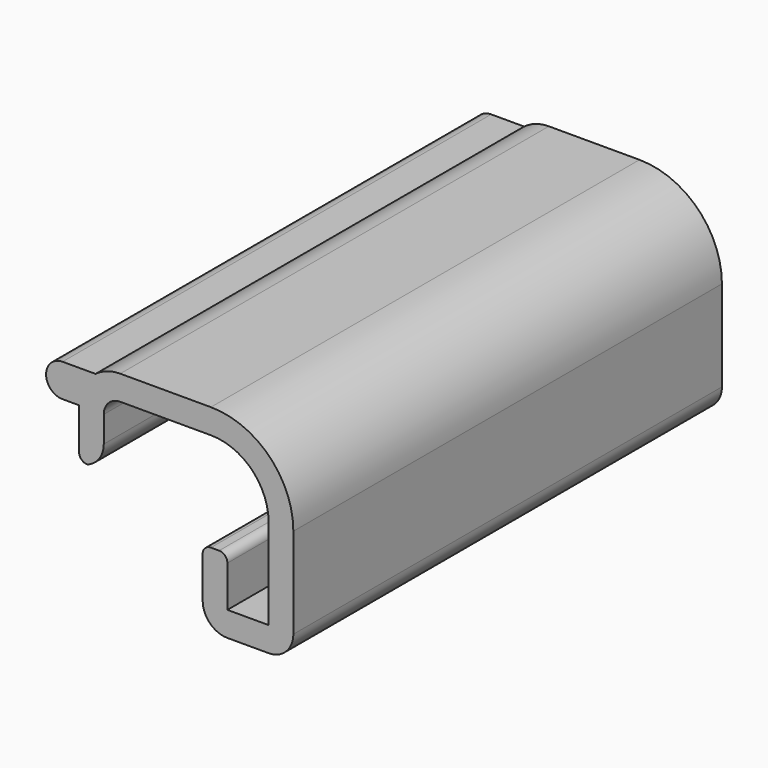
from build123d import *

# Parameters (mm, degrees)
F1_DEPTH    = 65
F2_R        = 1
F3_R        = 1.99999
F4_T1_DEPTH = 79.1421356237


# Not quite as in the source:
# - a fillet or chamfer that OpenCascade refuses, or shapes differently, is made with other operations: its cross-section is extruded or revolved along the edge and cut away or added
# - a fillet or chamfer is up to 0.001 mm smaller than in the source, because OpenCascade refuses the exact size
# - a feature names something its author has since deleted; it is built from what else it names


with BuildPart() as f1:
    # F0 (on Front) → F1 (new body)
    with BuildSketch(Plane.XZ):
        with BuildLine():
            ThreePointArc((0, -2), (0.5857864376, -0.5857864376), (2, 0))
            Line((2, 0), (13, 0))
            ThreePointArc((13, 0), (17.9497474683, -2.0502525317), (20, -7))
            Line((20, -7), (20, -18))
            Line((20, -18), (15, -18))
            Line((15, -18), (15, -12))
            Line((15, -12), (12, -12))
            Line((12, -12), (12, -18))
            ThreePointArc((12, -18), (12.8786796564, -20.1213203436), (15, -21))
            Line((15, -21), (20, -21))
            ThreePointArc((20, -21), (22.1213203436, -20.1213203436), (23, -18))
            Line((23, -18), (23, -7))
            ThreePointArc((23, -7), (20.0710678119, 0.0710678119), (13, 3))
            Line((13, 3), (2, 3))
            ThreePointArc((2, 3), (0.4188611699, 2.7434164903), (-1, 2))
            ThreePointArc((-1, 2), (-2.472135955, 0.2360679775), (-3, -2))
            Line((-3, -2), (-3, -8))
            Line((-3, -8), (0, -8))
            Line((0, -8), (0, -2))
        make_face()
        with BuildLine():
            Line((-7, -2), (-3, -2))
            ThreePointArc((-3, -2), (-2.472135955, 0.2360679775), (-1, 2))
            Line((-1, 2), (-7, 2))
            Line((-7, 2), (-7, -2))
        make_face()
    extrude(amount=F1_DEPTH)

    # F2
    f2_edges = [f1.edges().sort_by_distance(p)[0] for p in [
        (-3, -32.5, -8),
        (12, -32.5, -12),
        (15, -32.5, -12),
    ]]
    fillet(f2_edges, radius=F2_R)

    # F3 (radius 2 in the source; OpenCascade refuses exactly that, so slightly less here)
    f3_edges = [f1.edges().sort_by_distance(p)[0] for p in [
        (-7, -32.5, -2),
        (-7, -32.5, 2),
    ]]
    fillet(f3_edges, radius=F3_R)

    # F4: fillet of radius 3 on 1 edges, made by hand

    # F4_s2 → F4_t1 (cut)
    with BuildSketch(Plane.XZ.offset(-7.0710678119)):
        with BuildLine():
            ThreePointArc((-2, -8), (-0.5505102572, -6.9036236828), (0, -5.1715728753))
            Line((0, -5.1715728753), (0.06, -5.1715728753))
            Line((0.06, -5.1715728753), (0.06, -8))
            Line((0.06, -8), (0, -8.06))
            ThreePointArc((0, -8.06), (-1, -8.06), (-1.98, -8.0565685425))
            Line((-1.98, -8.0565685425), (-2, -8))
        make_face()
    extrude(amount=F4_T1_DEPTH, mode=Mode.SUBTRACT)


solid = f1.part
